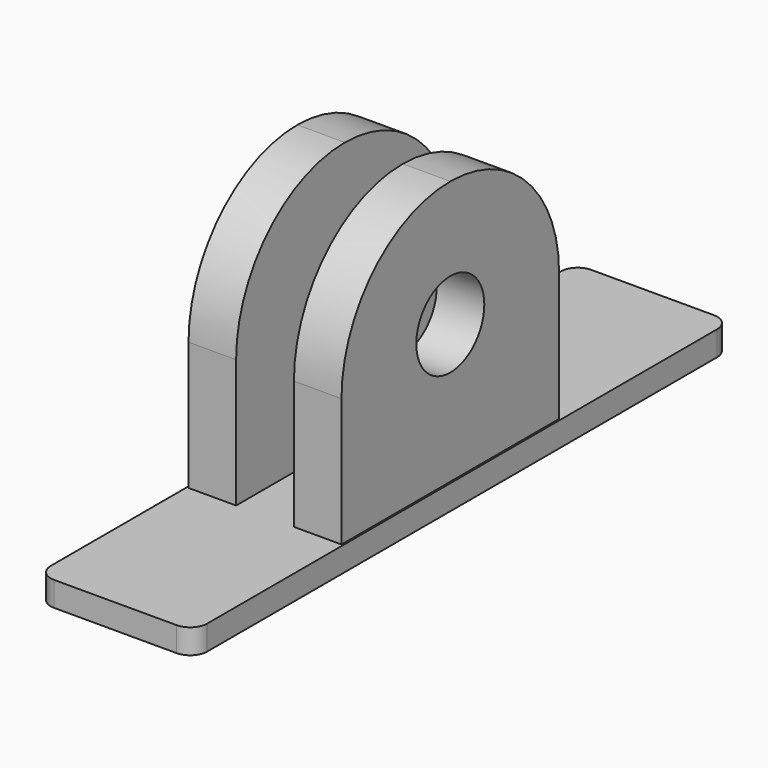
from build123d import *

# Parameters (mm, degrees)
F0_W     = 9.2
F0_H     = 39.5
F0_W_2   = 2.8
F0_H_2   = 16
F1_DEPTH = 1.45
F2_DEPTH = 17
F3_R     = 7.99999
F4_R     = 2.5
F5_DEPTH = 25
F6_R     = 1


# Not quite as in the source:
# - a fillet or chamfer is up to 0.001 mm smaller than in the source, because OpenCascade refuses the exact size


with BuildPart() as f1:
    # F0 (on Top) → F1 (new body)
    with BuildSketch(Plane.XY):
        with Locations((0.1172406439, 4.75)):
            Rectangle(F0_W, F0_H)
        with Locations((-2.9827593561, 4)):
            Rectangle(F0_W_2, F0_H_2, mode=Mode.SUBTRACT)
        with Locations((3.2172406439, 4)):
            Rectangle(F0_W_2, F0_H_2, mode=Mode.SUBTRACT)
    extrude(amount=F1_DEPTH)

    # F0 (on Top) → F2 (join)
    with BuildSketch(Plane.XY):
        with Locations((-2.9827593561, 4)):
            Rectangle(F0_W_2, F0_H_2)
        with Locations((3.2172406439, 4)):
            Rectangle(F0_W_2, F0_H_2)
    extrude(amount=F2_DEPTH)

    # F3 (radius 8 in the source; OpenCascade refuses exactly that, so slightly less here)
    f3_edges = [f1.edges().sort_by_distance(p)[0] for p in [
        (-2.982759, 12, 17),
        (3.217241, 12, 17),
        (3.217241, -4, 17),
        (-2.982759, -4, 17),
    ]]
    fillet(f3_edges, radius=F3_R)

    # F4 (on face) → F5 (cut)
    with BuildSketch(Plane.YZ.offset(4.6172406439)):
        with Locations((4, 9.6)):
            Circle(F4_R)
    extrude(amount=-F5_DEPTH, mode=Mode.SUBTRACT)

    # F6
    f6_edges = [f1.edges().sort_by_distance(p)[0] for p in [
        (4.717241, 24.5, 0.725),
        (-4.482759, 24.5, 0.725),
        (4.717241, -15, 0.725),
        (-4.482759, -15, 0.725),
    ]]
    fillet(f6_edges, radius=F6_R)


solid = f1.part
